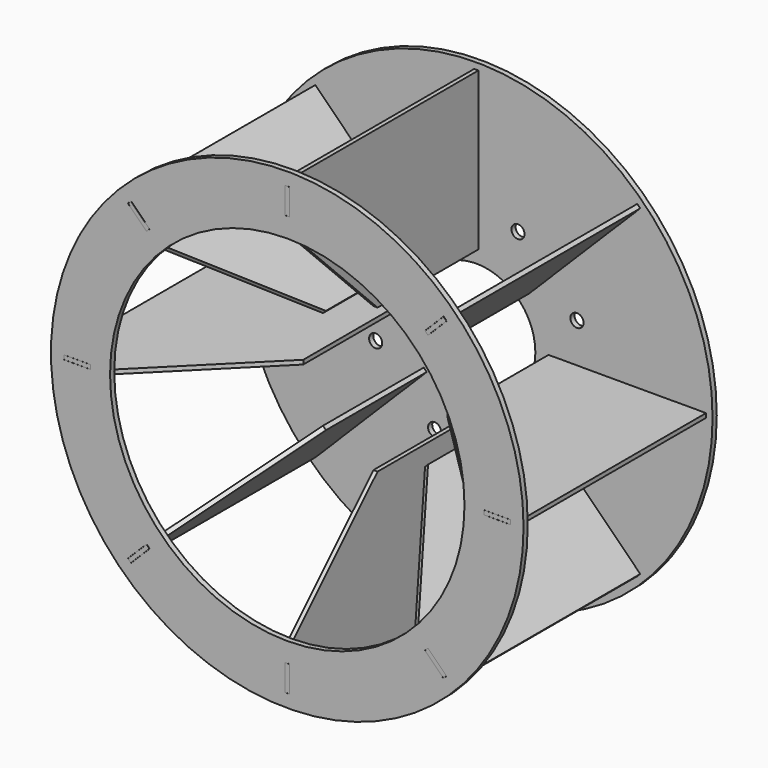
from build123d import *

# Parameters (mm, degrees)
F0_R          = 90
F0_R_2        = 22.5
F1_DEPTH      = 2
F3_R          = 2.5
F4_DEPTH      = 2.001
F5_W          = 1.65
F5_H          = 10
F5_W_2        = 10
F5_H_2        = 1.65
F6_DEPTH      = 2
F7_W          = 2
F7_H          = 10
F7_H_2        = 9.9
F8_DEPTH      = 0.8
F8_DEPTH_BACK = 0.8
F9_SIZE       = 40
F11_COUNT     = 8
F12_R         = 90
F12_W         = 1.64
F12_H         = 10.04
F12_W_2       = 10.04
F12_H_2       = 1.64
F12_R_2       = 67.5047405743
F13_DEPTH     = 2


# Not quite as in the source:
# - a feature names something its author has since deleted; it is built from what else it names


with BuildPart() as f1:
    # F0 (on Front) → F1 (new body)
    with BuildSketch(Plane.XZ):
        Circle(F0_R)
        Circle(F0_R_2, mode=Mode.SUBTRACT)
    extrude(amount=F1_DEPTH)

    # F3 (on face) → F4 (cut, through all)
    with BuildSketch(Plane.XZ.offset(2)):
        with Locations((15.8813624432, 38.3410005992)):
            Circle(F3_R)
        with Locations((-15.8813624432, 38.3410005992)):
            Circle(F3_R)
        with Locations((-38.3410005992, 15.8813624432)):
            Circle(F3_R)
        with Locations((-38.3410005992, -15.8813624432)):
            Circle(F3_R)
        with Locations((-15.8813624432, -38.3410005992)):
            Circle(F3_R)
        with Locations((15.8813624432, -38.3410005992)):
            Circle(F3_R)
        with Locations((38.3410005992, -15.8813624432)):
            Circle(F3_R)
        with Locations((38.3410005992, 15.8813624432)):
            Circle(F3_R)
    extrude(amount=-F4_DEPTH, mode=Mode.SUBTRACT)

    # F5 (on face) → F6 (cut, through all)
    with BuildSketch(Plane.XZ.offset(2)):
        with Locations((0, 80)):
            Rectangle(F5_W, F5_H)
        with Locations((0, 35)):
            Rectangle(F5_W, F5_H)
        Polygon((-52.4496454945, 53.6163716835), (-59.5207133064, 60.6874394953), (-60.6874394953, 59.5207133064), (-53.6163716835, 52.4496454945), align=None)
        Polygon((-20.6298403411, 21.7965665301), (-27.700908153, 28.8676343419), (-28.8676343419, 27.700908153), (-21.7965665301, 20.6298403411), align=None)
        with Locations((-80, 0)):
            Rectangle(F5_W_2, F5_H_2)
        with Locations((-35, 0)):
            Rectangle(F5_W_2, F5_H_2)
        Polygon((-53.6163716835, -52.4496454945), (-60.6874394953, -59.5207133064), (-59.5207133064, -60.6874394953), (-52.4496454945, -53.6163716835), align=None)
        Polygon((-21.7965665301, -20.6298403411), (-28.8676343419, -27.700908153), (-27.700908153, -28.8676343419), (-20.6298403411, -21.7965665301), align=None)
        with Locations((0, -80)):
            Rectangle(F5_W, F5_H)
        with Locations((0, -35)):
            Rectangle(F5_W, F5_H)
        Polygon((52.4496454945, -53.6163716835), (59.5207133064, -60.6874394953), (60.6874394953, -59.5207133064), (53.6163716835, -52.4496454945), align=None)
        Polygon((20.6298403411, -21.7965665301), (27.700908153, -28.8676343419), (28.8676343419, -27.700908153), (21.7965665301, -20.6298403411), align=None)
        with Locations((80, 0)):
            Rectangle(F5_W_2, F5_H_2)
        with Locations((35, 0)):
            Rectangle(F5_W_2, F5_H_2)
        Polygon((53.6163716835, 52.4496454945), (60.6874394953, 59.5207133064), (59.5207133064, 60.6874394953), (52.4496454945, 53.6163716835), align=None)
        Polygon((21.7965665301, 20.6298403411), (28.8676343419, 27.700908153), (27.700908153, 28.8676343419), (20.6298403411, 21.7965665301), align=None)
    extrude(amount=-F6_DEPTH, mode=Mode.SUBTRACT)


with BuildPart() as f8:
    # F7 (on Right) → F8 (new body, two sides)
    with BuildSketch(Plane.YZ) as f8_sk:
        Polygon((-2, 87.5), (-90, 87.5), (-90, 85), (-90, 75), (-90, 27.5), (-2, 27.5), (-2, 30.05), (-2, 39.95), (-2, 75.05), (-2, 84.95), align=None)
        with Locations((-91, 80)):
            Rectangle(F7_W, F7_H)
        with Locations((-1, 80)):
            Rectangle(F7_W, F7_H_2)
        with Locations((-1, 35)):
            Rectangle(F7_W, F7_H_2)
    extrude(amount=F8_DEPTH)
    extrude(f8_sk.sketch, amount=-F8_DEPTH_BACK)

    # F9
    f9_edges = [f8.edges().sort_by_distance(p)[0] for p in [
        (0, -90, 27.5),
    ]]
    chamfer(f9_edges, length=F9_SIZE)


with BuildPart() as f11_1:
    # F11: instance of F8
    add(f8.part.rotate(Axis((0, -63.7029781938, 0), (0, -1, 0)), 1 * 360 / F11_COUNT))


with BuildPart() as f11_2:
    # F11: instance of F8
    add(f8.part.rotate(Axis((0, -63.7029781938, 0), (0, -1, 0)), 2 * 360 / F11_COUNT))


with BuildPart() as f11_3:
    # F11: instance of F8
    add(f8.part.rotate(Axis((0, -63.7029781938, 0), (0, -1, 0)), 3 * 360 / F11_COUNT))


with BuildPart() as f11_4:
    # F11: instance of F8
    add(f8.part.rotate(Axis((0, -63.7029781938, 0), (0, -1, 0)), 4 * 360 / F11_COUNT))


with BuildPart() as f11_5:
    # F11: instance of F8
    add(f8.part.rotate(Axis((0, -63.7029781938, 0), (0, -1, 0)), 5 * 360 / F11_COUNT))


with BuildPart() as f11_6:
    # F11: instance of F8
    add(f8.part.rotate(Axis((0, -63.7029781938, 0), (0, -1, 0)), 6 * 360 / F11_COUNT))


with BuildPart() as f11_7:
    # F11: instance of F8
    add(f8.part.rotate(Axis((0, -63.7029781938, 0), (0, -1, 0)), 7 * 360 / F11_COUNT))


with BuildPart() as f13:
    # F12 (on face) → F13 (new body)
    with BuildSketch(Plane.XZ.offset(90)):
        Circle(F12_R)
        Polygon((-60.6980460971, -59.5383909759), (-53.5986940139, -52.4390388928), (-52.4390388928, -53.5986940139), (-59.5383909759, -60.6980460971), align=None, mode=Mode.SUBTRACT)
        with Locations((0, -80)):
            Rectangle(F12_W, F12_H, mode=Mode.SUBTRACT)
        Polygon((59.5383909759, -60.6980460971), (52.4390388928, -53.5986940139), (53.5986940139, -52.4390388928), (60.6980460971, -59.5383909759), align=None, mode=Mode.SUBTRACT)
        with Locations((-80, 0)):
            Rectangle(F12_W_2, F12_H_2, mode=Mode.SUBTRACT)
        Polygon((-59.5383909759, 60.6980460971), (-52.4390388928, 53.5986940139), (-53.5986940139, 52.4390388928), (-60.6980460971, 59.5383909759), align=None, mode=Mode.SUBTRACT)
        Circle(F12_R_2, mode=Mode.SUBTRACT)
        with Locations((80, 0)):
            Rectangle(F12_W_2, F12_H_2, mode=Mode.SUBTRACT)
        with Locations((0, 80)):
            Rectangle(F12_W, F12_H, mode=Mode.SUBTRACT)
        Polygon((60.6980460971, 59.5383909759), (53.5986940139, 52.4390388928), (52.4390388928, 53.5986940139), (59.5383909759, 60.6980460971), align=None, mode=Mode.SUBTRACT)
    extrude(amount=F13_DEPTH)


solid = Compound([f1.part, f8.part, f11_1.part, f11_2.part, f11_3.part, f11_4.part, f11_5.part, f11_6.part, f11_7.part, f13.part])
